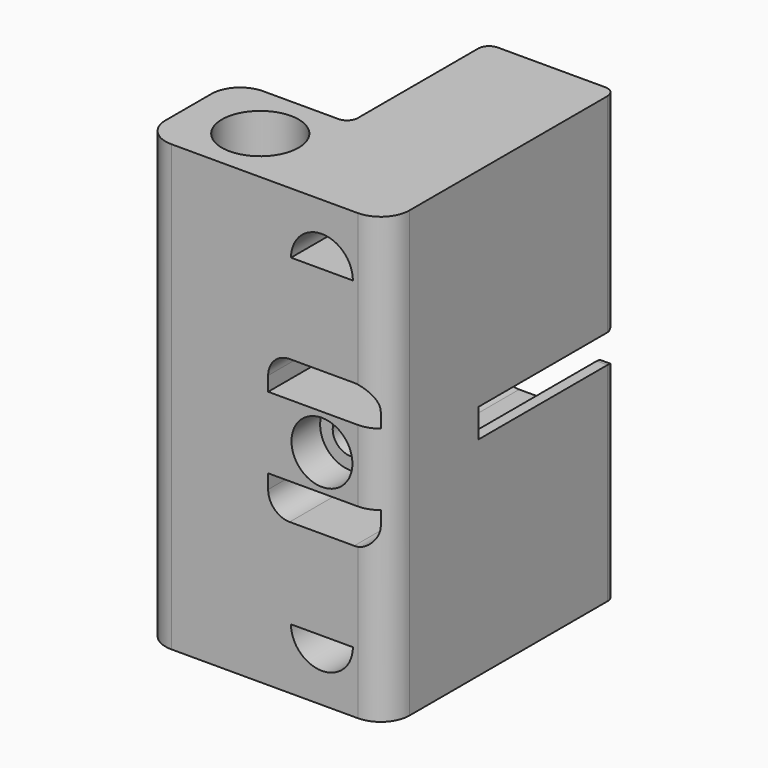
from build123d import *

# Parameters (mm, degrees)
F0_W            = 18
F0_H            = 62
F0_R            = 4.315
F1_DEPTH        = 40
F3_DEPTH        = 16
F4_R            = 5.35
F5_DEPTH        = 100
F6_R            = 1.5625
F6_R_2          = 5.375
F7_DEPTH        = 10
F8_DEPTH        = 10
F10_DEPTH       = 100
F9_W            = 1.5
F9_H            = 2
F11_DEPTH       = 24
F12_W           = 15
F12_H           = 10
F13_DEPTH       = 8
F14_SIZE2       = 3
F14_SIZE        = 1
F14_2_SIZE2     = 3
F14_2_SIZE      = 1
F15_R           = 3
F16_T1_DEPTH    = 62
F16_T3_DEPTH    = 82
F16_T5_DEPTH    = 30
F17_R           = 1.49999
F18_D           = 5
F18_DEPTH       = 10
F18_CBORE_D     = 8.5
F18_CBORE_DEPTH = 5
F18_TIP         = 1.5021515476


# Not quite as in the source:
# - a fillet or chamfer that OpenCascade refuses, or shapes differently, is made with other operations: its cross-section is extruded or revolved along the edge and cut away or added
# - a fillet or chamfer is up to 0.001 mm smaller than in the source, because OpenCascade refuses the exact size


with BuildPart() as f1:
    # F0 (on Front) → F1 (new body)
    with BuildSketch(Plane.XZ):
        Rectangle(F0_W, F0_H)
        with Locations((0, -22.5)):
            Circle(F0_R, mode=Mode.SUBTRACT)
        with Locations((0, 22.5)):
            Circle(F0_R, mode=Mode.SUBTRACT)
    extrude(amount=F1_DEPTH)

    # F2 (on face) → F3 (join)
    with BuildSketch(Plane(origin=(-9, 0, 0), x_dir=(0, -1, 0), z_dir=(-1, 0, 0))):
        Polygon((24, 31), (24, 0), (24, -31), (40, -31), (40, 31), align=None)
    extrude(amount=F3_DEPTH)

    # F4 (on face) → F5 (cut)
    with BuildSketch(Plane(origin=(0, 0, -31), x_dir=(1, 0, 0), z_dir=(0, 0, -1))):
        with Locations((-15, 32)):
            Circle(F4_R)
    extrude(amount=-F5_DEPTH, mode=Mode.SUBTRACT)

    # F6 (on face) → F7 (join)
    with BuildSketch(Plane(origin=(0, 0, -31), x_dir=(1, 0, 0), z_dir=(0, 0, -1))):
        with BuildLine():
            Line((-9, 22.2923703349), (-9, 24))
            Line((-9, 24), (-25, 24))
            Line((-25, 24), (-25, 6.5))
            Line((-25, 6.5), (-9, 6.5))
            Line((-9, 6.5), (-9, 7.7076296651))
            ThreePointArc((-9, 7.7076296651), (-10.8125, 9.25), (-9, 10.7923703349))
            Line((-9, 10.7923703349), (-9, 19.2076296651))
            ThreePointArc((-9, 19.2076296651), (-10.8125, 20.75), (-9, 22.2923703349))
        make_face()
        with Locations((-20.75, 9.25)):
            Circle(F6_R, mode=Mode.SUBTRACT)
        with Locations((-15, 15)):
            Circle(F6_R_2, mode=Mode.SUBTRACT)
        with Locations((-20.75, 20.75)):
            Circle(F6_R, mode=Mode.SUBTRACT)
    extrude(amount=-F7_DEPTH)

    # F6 (on face) → F8 (cut)
    with BuildSketch(Plane(origin=(0, 0, -31), x_dir=(1, 0, 0), z_dir=(0, 0, -1))):
        with BuildLine():
            ThreePointArc((-7.6875, 20.75), (-8.0600354522, 21.7626157341), (-9, 22.2923703349))
            Line((-9, 22.2923703349), (-9, 19.2076296651))
            ThreePointArc((-9, 19.2076296651), (-8.0600354522, 19.7373842659), (-7.6875, 20.75))
        make_face()
        with BuildLine():
            ThreePointArc((-7.6875, 9.25), (-8.0600354522, 10.2626157341), (-9, 10.7923703349))
            Line((-9, 10.7923703349), (-9, 7.7076296651))
            ThreePointArc((-9, 7.7076296651), (-8.0600354522, 8.2373842659), (-7.6875, 9.25))
        make_face()
    extrude(amount=-F8_DEPTH, mode=Mode.SUBTRACT)

    # F9 (on face) → F10 (cut)
    with BuildSketch(Plane(origin=(0, 0, 0), x_dir=(-1, 0, 0), z_dir=(0, 1, 0))):
        Polygon((7.5, 2), (7.5, 10), (-7.5, 10), (-7.5, 2), (-7.5, 0), (0, 0), (7.5, 0), align=None)
        Polygon((7.5, -2), (7.5, 0), (0, 0), (-7.5, 0), (-7.5, -2), (-7.5, -10), (7.5, -10), align=None)
    extrude(amount=-F10_DEPTH, mode=Mode.SUBTRACT)

    # F9 (on face) → F11 (cut)
    with BuildSketch(Plane(origin=(0, 0, 0), x_dir=(-1, 0, 0), z_dir=(0, 1, 0))):
        with Locations((-8.25, -1)):
            Rectangle(F9_W, F9_H)
        with Locations((-8.25, 1)):
            Rectangle(F9_W, F9_H)
        with Locations((8.25, -1)):
            Rectangle(F9_W, F9_H)
        with Locations((8.25, 1)):
            Rectangle(F9_W, F9_H)
    extrude(amount=-F11_DEPTH, mode=Mode.SUBTRACT)

    # F12 (on face) → F13 (join)
    with BuildSketch(Plane.XZ.offset(40)):
        Rectangle(F12_W, F12_H)
        with BuildLine():
            Line((4.315, 22.5), (0, 22.5))
            Line((0, 22.5), (-4.315, 22.5))
            ThreePointArc((-4.315, 22.5), (0, 18.185), (4.315, 22.5))
        make_face()
        with BuildLine():
            Line((-4.315, -22.5), (0, -22.5))
            Line((0, -22.5), (4.315, -22.5))
            ThreePointArc((4.315, -22.5), (0, -18.185), (-4.315, -22.5))
        make_face()
    extrude(amount=-F13_DEPTH)

    # F14
    f14_edges = [f1.edges().sort_by_distance(p)[0] for p in [
        (-4.315, 0, 22.5),
    ]]
    f14_side = f1.faces().sort_by_distance((8.25, 0, 2.341321))[0]
    chamfer(f14_edges, length=F14_SIZE, length2=F14_SIZE2, reference=f14_side)

    # F14#2
    f14_2_edges = [f1.edges().sort_by_distance(p)[0] for p in [
        (-4.315, 0, -22.5),
    ]]
    f14_2_side = f1.faces().sort_by_distance((0, 0, -30.658679))[0]
    chamfer(f14_2_edges, length=F14_2_SIZE, length2=F14_2_SIZE2, reference=f14_2_side)

    # F15
    f15_edges = [f1.edges().sort_by_distance(p)[0] for p in [
        (-7.5, -20, 10),
        (7.5, -20, 10),
        (7.5, -20, -10),
        (-7.5, -20, -10),
    ]]
    fillet(f15_edges, radius=F15_R)

    # F16: fillet of radius 4 on 4 edges, made by hand

    # F16_s2 → F16_t1 (cut)
    with BuildSketch(Plane.XY.offset(-21)):
        with BuildLine():
            ThreePointArc((-21, -24), (-23.8284271247, -25.1715728753), (-25, -28))
            Line((-25, -28), (-25, -24))
            Line((-25, -24), (-21, -24))
        make_face()
    extrude(amount=F16_T1_DEPTH, mode=Mode.SUBTRACT)

    # F16_s4 → F16_t3 (cut)
    with BuildSketch(Plane.XY.offset(-41)):
        with BuildLine():
            ThreePointArc((-21, -40), (-23.8284271247, -38.8284271247), (-25, -36))
            Line((-25, -36), (-25, -40))
            Line((-25, -40), (-21, -40))
        make_face()
        with BuildLine():
            ThreePointArc((9, -36), (7.8284271247, -38.8284271247), (5, -40))
            Line((5, -40), (9, -40))
            Line((9, -40), (9, -36))
        make_face()
    extrude(amount=F16_T3_DEPTH, mode=Mode.SUBTRACT)

    # F16_s6 → F16_t5 (cut)
    with BuildSketch(Plane.XY.offset(-41)):
        with BuildLine():
            ThreePointArc((-21, -6.5), (-23.8284271247, -7.6715728753), (-25, -10.5))
            Line((-25, -10.5), (-25, -6.5))
            Line((-25, -6.5), (-21, -6.5))
        make_face()
    extrude(amount=F16_T5_DEPTH, mode=Mode.SUBTRACT)

    # F17 (radius 1.5 in the source; OpenCascade refuses exactly that, so slightly less here)
    f17_edges = [f1.edges().sort_by_distance(p)[0] for p in [
        (-25, -10.5, -26),
        (-9, 0, -16.5),
        (9, 0, -16.5),
        (-9, -24, -11.5),
        (-9, -24, 16.5),
        (9, 0, 16.5),
        (-9, 0, 16.5),
        (-8.25, 0, 2),
        (-8.25, 0, -2),
        (8.25, 0, -2),
        (8.25, 0, 2),
    ]]
    fillet(f17_edges, radius=F17_R)

    # F18
    with Locations(Plane.XZ.offset(40)):
        with Locations((0, 0)):
            CounterBoreHole(F18_D / 2, F18_CBORE_D / 2, F18_CBORE_DEPTH, depth=F18_DEPTH)
            with Locations((0, 0, -(F18_DEPTH + F18_TIP / 2))):  # 118° drill point
                Cone(0, F18_D / 2, F18_TIP, mode=Mode.SUBTRACT)


solid = f1.part
